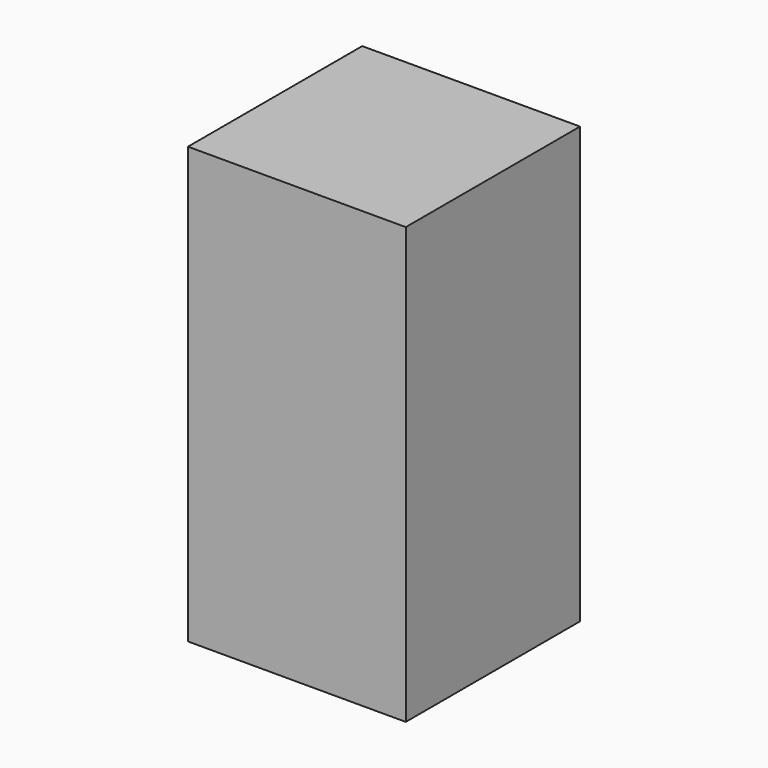
from build123d import *

# Parameters (mm, degrees)
F1_W     = 76.2
F1_H     = 152.4
F2_DEPTH = 38.1


# Not quite as in the source:
# - a variable given as a bare number and used for a length is read in inches; the dataset says mm whatever the document's units were


with BuildPart() as f2:
    # F1 (on Front) → F2 (new body, symmetric)
    with BuildSketch(Plane.XZ):
        Rectangle(F1_W, F1_H)
    extrude(amount=F2_DEPTH, both=True)


solid = f2.part
